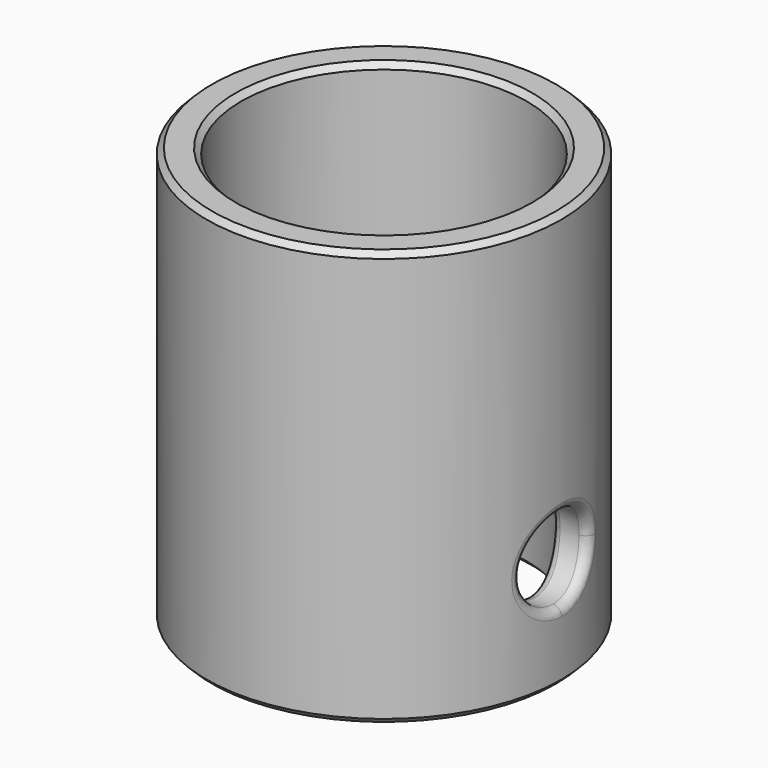
from build123d import *

# Parameters (mm, degrees)
F0_R     = 6.4
F0_R_2   = 5.15
F1_DEPTH = 15
F2_R     = 1.5
F3_DEPTH = 275
F4_R     = 0.3
F5_SIZE  = 0.2


with BuildPart() as f1:
    # F0 (on Top) → F1 (new body)
    with BuildSketch(Plane.XY):
        Circle(F0_R)
        Circle(F0_R_2, mode=Mode.SUBTRACT)
    extrude(amount=F1_DEPTH)

    # F2 (on Right) → F3 (cut, symmetric)
    with BuildSketch(Plane.YZ):
        with Locations((0, 4)):
            Circle(F2_R)
    extrude(amount=F3_DEPTH, both=True, mode=Mode.SUBTRACT)

    # F4
    f4_edges = [f1.edges().sort_by_distance(p)[0] for p in [
        (6.221736, -1.5, 4),
        (6.311492, 1.060695, 5.060625),
        (6.311492, 1.060695, 2.939375),
        (-6.221736, -1.5, 4),
        (4.926713, -1.5, 4),
        (5.039575, 1.060745, 5.060575),
        (5.039575, 1.060745, 2.939425),
        (-4.926713, -1.5, 4),
    ]]
    fillet(f4_edges, radius=F4_R)

    # F5
    f5_edges = [f1.edges().sort_by_distance(p)[0] for p in [
        (-6.4, 0, 15),
        (-5.15, 0, 15),
        (-6.4, 0, 0),
        (-5.15, 0, 0),
    ]]
    chamfer(f5_edges, length=F5_SIZE)


solid = f1.part
